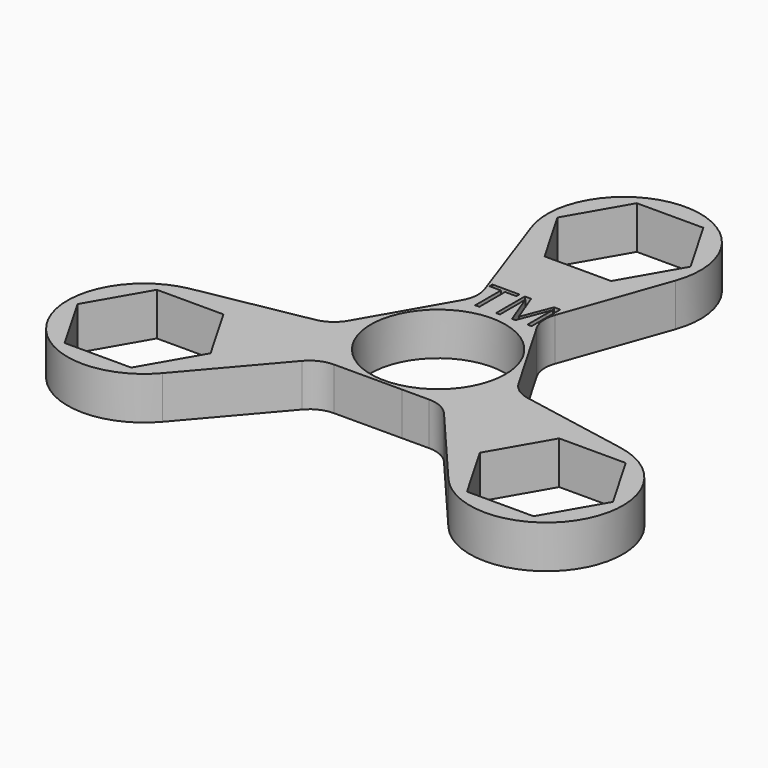
from build123d import *

# Parameters (mm, degrees)
F0_R         = 11
F1_DEPTH     = 7
F3_DEPTH     = 25
F4_R         = 5
F5_TEXT_SIZE = 8.2102591804
F6_DEPTH     = 3


# Not quite as in the source:
# - Text() gives the source's letters only with a copy of the font that has no kerning and outlines rounded to 1/6400 em; it was checked with that copy


with BuildPart() as f1:
    # F0 (on Top) → F1 (new body)
    with BuildSketch(Plane.XY):
        with BuildLine():
            Line((4.9421419792, 14.5017044169), (11.7795150754, 33.7585096458))
            ThreePointArc((11.7795150754, 33.7585096458), (0.0125756633, 50.4409696484), (-11.7879067922, 33.7822197348))
            Line((-11.7879067922, 33.7822197348), (-4.9857692462, 14.5017044169))
            Line((-4.9857692462, 14.5017044169), (-15.0299154128, -2.9708317054))
            Line((-15.0299154128, -2.9708317054), (-35.1254844849, -6.6778955234))
            ThreePointArc((-35.1254844849, -6.6778955234), (-43.6894489387, -25.2095939803), (-23.3623070905, -27.0997366068))
            Line((-23.3623070905, -27.0997366068), (-10.0659598001, -11.5686550331))
            Line((-10.0659598001, -11.5686550331), (3.3500355549, -11.5435039882))
            Line((3.3500355549, -11.5435039882), (10.0877734337, -11.5308727115))
            Line((10.0877734337, -11.5308727115), (23.3459694095, -27.0806141225))
            ThreePointArc((23.3459694095, -27.0806141225), (43.6768732754, -25.2313756681), (35.1502138826, -6.6824831279))
            Line((35.1502138826, -6.6824831279), (15.0517290464, -2.9330493838))
            Line((15.0517290464, -2.9330493838), (14.8760446113, -2.6300681788))
            Line((14.8760446113, -2.6300681788), (4.9421419792, 14.5017044169))
        make_face()
        Circle(F0_R, mode=Mode.SUBTRACT)
    extrude(amount=F1_DEPTH)

    # F2 (on face) → F3 (cut)
    with BuildSketch(Plane.XY.offset(7)):
        Polygon((5.4357527844, 47.3559759743), (-5.4357527844, 47.3559759743), (-10.8715055688, 37.9409759743), (-5.4357527844, 28.5259759743), (5.4357527844, 28.5259759743), (10.8715055688, 37.9409759743), align=None)
        Polygon((-43.7293546069, -18.9704879871), (-38.2936018225, -28.3854879871), (-27.4220962537, -28.3854879871), (-21.9863434693, -18.9704879871), (-27.4220962537, -9.5554879871), (-38.2936018225, -9.5554879871), align=None)
        Polygon((38.2936018225, -28.3854879871), (43.7293546069, -18.9704879871), (38.2936018225, -9.5554879871), (27.4220962537, -9.5554879871), (21.9863434693, -18.9704879871), (27.4220962537, -28.3854879871), align=None)
    extrude(amount=-F3_DEPTH, mode=Mode.SUBTRACT)

    # F4
    f4_edges = [f1.edges().sort_by_distance(p)[0] for p in [
        (10.087773, -11.530873, 3.5),
        (-10.06596, -11.568655, 3.5),
        (4.942142, 14.501704, 3.5),
        (-15.029915, -2.970832, 3.5),
        (-4.985769, 14.501704, 3.5),
        (15.051729, -2.933049, 3.5),
    ]]
    fillet(f4_edges, radius=F4_R)

    # F5 (on face) → F6 (cut)
    with BuildSketch(Plane.XY.offset(7)):
        with Locations((-5.8427539745, 12.4564114831)):
            Text('TM', F5_TEXT_SIZE, font='Open Sans', text_align=(TextAlign.LEFT, TextAlign.BOTTOM))
    extrude(amount=-F6_DEPTH, mode=Mode.SUBTRACT)


solid = f1.part
